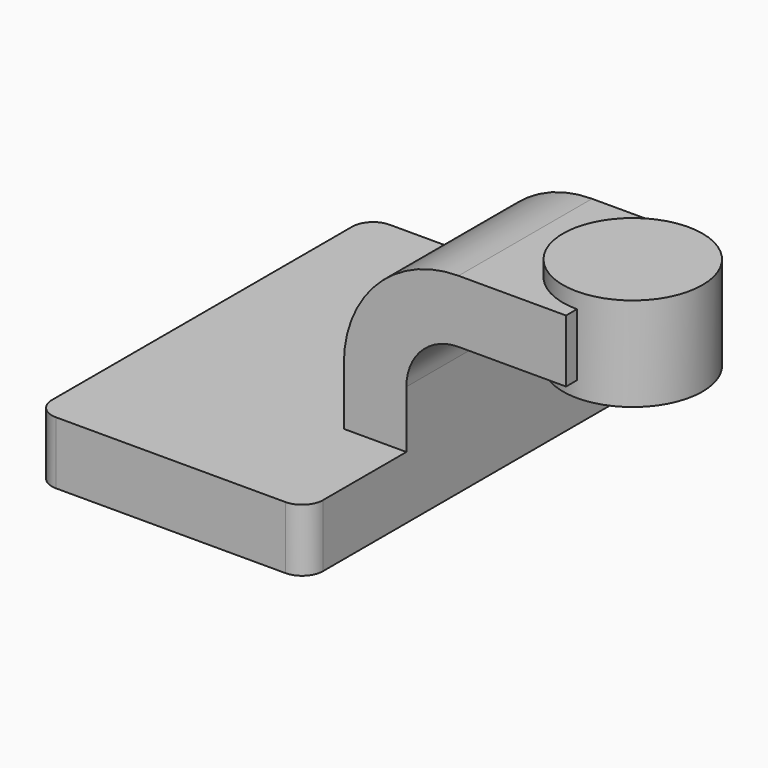
from build123d import *

# Parameters (mm, degrees)
F1_DEPTH = 63.5
F0_W     = 29.5617593795
F0_H     = 19.05
F2_DEPTH = 25.4
F5_R     = 6.35


# Not quite as in the source:
# - a feature of the source that left no trace in its solid (it failed there, or was rolled back) is left out


with BuildPart() as f1:
    # F0 (on Front) → F1 (new body, symmetric)
    with BuildSketch(Plane.XZ):
        Polygon((41.275, -9.525), (41.275, 9.525), (22.225, 9.525), (-41.275, 9.525), (-41.275, -9.525), align=None)
    extrude(amount=F1_DEPTH, both=True)

    # F0 (on Front) → F2 (join, symmetric)
    with BuildSketch(Plane.XZ):
        with BuildLine():
            Line((22.225, 9.525), (41.275, 9.525))
            Line((41.275, 9.525), (41.275, 27.0002))
            ThreePointArc((41.275, 27.0002), (45.9246798487, 38.2255201513), (57.15, 42.8752))
            Line((57.15, 42.8752), (60.325, 42.8752))
            Line((60.325, 42.8752), (60.325, 61.9252))
            Line((60.325, 61.9252), (57.15, 61.9252))
            ThreePointArc((57.15, 61.9252), (32.4542956671, 51.6959043329), (22.225, 27.0002))
            Line((22.225, 27.0002), (22.225, 9.525))
        make_face()
        with Locations((75.1058796897, 52.4002)):
            Rectangle(F0_W, F0_H)
    extrude(amount=F2_DEPTH, both=True)

    # F0 (on Front) → F4 (revolve)
    with BuildSketch(Plane.XZ):
        Polygon((89.8867593795, 61.9252), (89.8867593795, 42.8752), (89.8867593795, 38.1), (111.125, 38.1), (111.125, 66.675), (89.8867593795, 66.675), align=None)
    revolve(axis=Axis((89.8867593795, 0, 52.3875), (0, 0, 1)))

    # F5
    f5_edges = [f1.edges().sort_by_distance(p)[0] for p in [
        (41.275, -63.5, 0),
        (-41.275, -63.5, 0),
        (41.275, 63.5, 0),
        (-41.275, 63.5, 0),
    ]]
    fillet(f5_edges, radius=F5_R)


solid = f1.part
